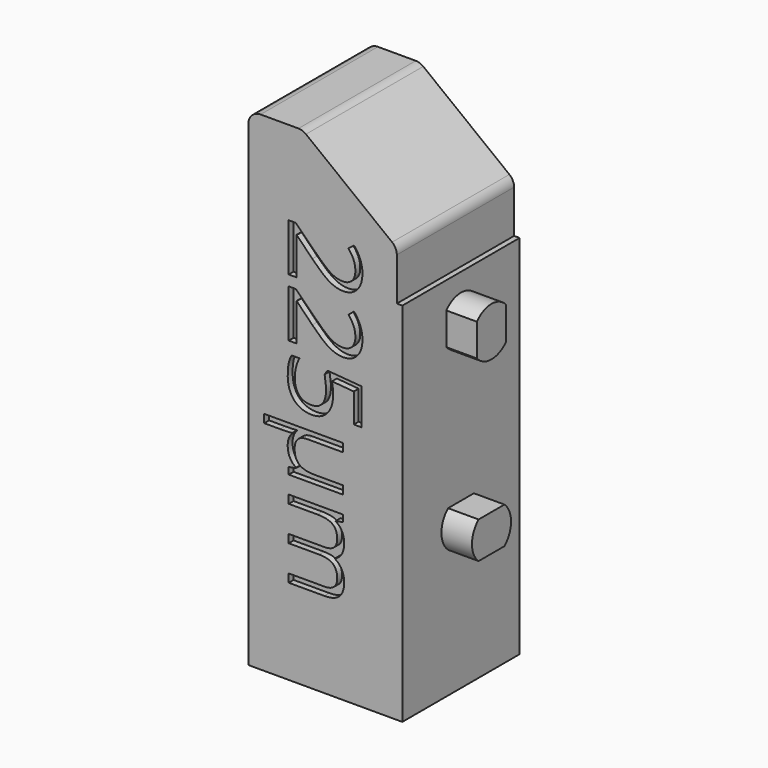
from build123d import *

# Parameters (mm, degrees)
F1_DEPTH     = 6
F3_DEPTH     = 1.25
F4_R         = 1.075
F5_DEPTH     = 5
F6_R         = 0.5
F7_TEXT_SIZE = 4.1666666667
F8_DEPTH     = 0.25


# Not quite as in the source:
# - Text() gives the source's letters only with a copy of the font that has no kerning and outlines rounded to 1/6400 em; it was checked with that copy


with BuildPart() as f1:
    # F0 (on Front) → F1 (new body)
    with BuildSketch(Plane.XZ):
        Polygon((2.925, 7), (-0.9286696865, 10), (-3.15, 10), (-3.15, -10), (3.15, -10), (3.15, 5), (2.925, 5), align=None)
    extrude(amount=F1_DEPTH)

    # F2 (on face) → F3 (join)
    with BuildSketch(Plane.YZ.offset(3.15)):
        with BuildLine():
            Line((-2.3385621722, -3.25), (-3.6614378278, -3.25))
            ThreePointArc((-3.6614378278, -3.25), (-4, -4), (-3.6614378278, -4.75))
            Line((-3.6614378278, -4.75), (-2.3385621722, -4.75))
            ThreePointArc((-2.3385621722, -4.75), (-2, -4), (-2.3385621722, -3.25))
        make_face()
        with BuildLine():
            Line((-3.75, 3.9114378278), (-3.75, 2.5885621722))
            ThreePointArc((-3.75, 2.5885621722), (-3, 2.25), (-2.25, 2.5885621722))
            Line((-2.25, 2.5885621722), (-2.25, 3.9114378278))
            ThreePointArc((-2.25, 3.9114378278), (-3, 4.25), (-3.75, 3.9114378278))
        make_face()
    extrude(amount=F3_DEPTH)

    # F4 (on face) → F5 (cut)
    with BuildSketch(Plane(origin=(0, 0, -10), x_dir=(1, 0, 0), z_dir=(0, 0, -1))):
        with Locations((-0.15, 3)):
            Circle(F4_R)
    extrude(amount=-F5_DEPTH, mode=Mode.SUBTRACT)

    # F6
    f6_edges = [f1.edges().sort_by_distance(p)[0] for p in [
        (2.925, -3, 7),
        (-0.92867, -3, 10),
        (-3.15, -3, 10),
    ]]
    fillet(f6_edges, radius=F6_R)

    # F7 (on face) → F8 (cut)
    with BuildSketch(Plane.XZ.offset(6)):
        with Locations(Location((-1.5, 6.7672526042), (0, 0, -90))):
            Text('225µm', F7_TEXT_SIZE, font='Open Sans', text_align=(TextAlign.LEFT, TextAlign.BOTTOM))
    extrude(amount=-F8_DEPTH, mode=Mode.SUBTRACT)


solid = f1.part
